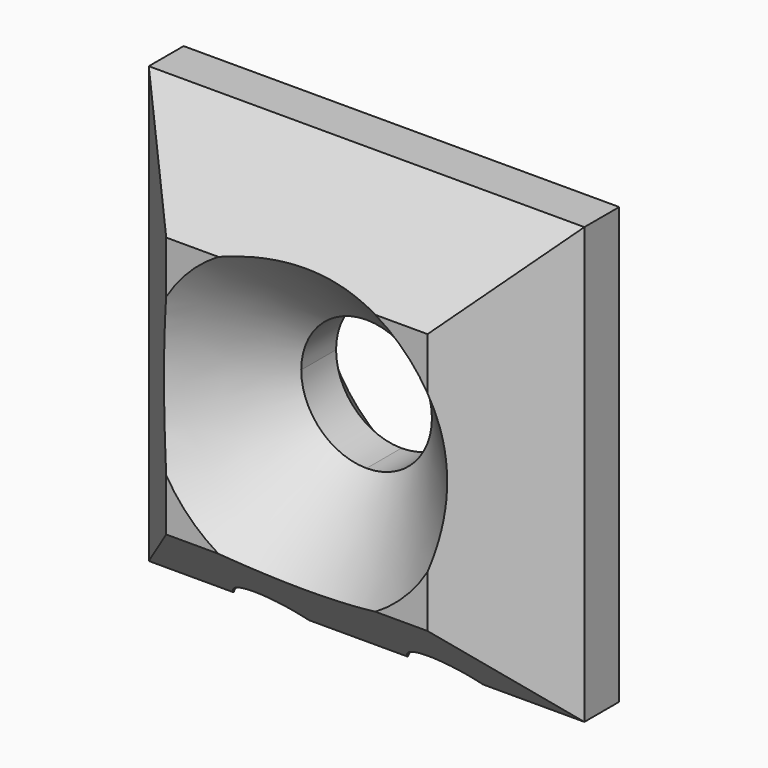
from build123d import *

# Parameters (mm, degrees)
F1_DEPTH    = 12.7
F2_R        = 2.54
F3_DEPTH    = 2.54
F4_T1_DEPTH = 51.5282991577
F4_T3_DEPTH = 51.5282991577


# Not quite as in the source:
# - a fillet or chamfer that OpenCascade refuses, or shapes differently, is made with other operations: its cross-section is extruded or revolved along the edge and cut away or added


with BuildPart() as f1:
    # F0 (on Front) → F1 (new body)
    with BuildSketch(Plane.XZ):
        with BuildLine():
            Line((0, 25.4), (0, 12.7))
            Line((0, 12.7), (8.89, 12.7))
            ThreePointArc((8.89, 12.7), (10.0059231637, 15.3940768363), (12.7, 16.51))
            Line((12.7, 16.51), (12.7, 25.4))
            Line((12.7, 25.4), (0, 25.4))
        make_face()
        with BuildLine():
            Line((16.51, 12.7), (25.4, 12.7))
            Line((25.4, 12.7), (25.4, 25.4))
            Line((25.4, 25.4), (12.7, 25.4))
            Line((12.7, 25.4), (12.7, 16.51))
            ThreePointArc((12.7, 16.51), (15.3940768363, 15.3940768363), (16.51, 12.7))
        make_face()
        with BuildLine():
            Line((12.7, 8.89), (12.7, 0))
            Line((12.7, 0), (25.4, 0))
            Line((25.4, 0), (25.4, 12.7))
            Line((25.4, 12.7), (16.51, 12.7))
            ThreePointArc((16.51, 12.7), (15.3940768363, 10.0059231637), (12.7, 8.89))
        make_face()
        with BuildLine():
            Line((0, 12.7), (0, 0))
            Line((0, 0), (12.7, 0))
            Line((12.7, 0), (12.7, 8.89))
            ThreePointArc((12.7, 8.89), (10.0059231637, 10.0059231637), (8.89, 12.7))
            Line((8.89, 12.7), (0, 12.7))
        make_face()
    extrude(amount=F1_DEPTH)

    # F2 (on Top) → F3 (cut)
    with BuildSketch(Plane.XY):
        with Locations((7.1409146445, -6.35)):
            Circle(F2_R)
        with Locations((17.3009146445, -6.35)):
            Circle(F2_R)
    extrude(amount=F3_DEPTH, mode=Mode.SUBTRACT)

    # F4: chamfer of 5.08 on 10 edges, made by hand

    # F4_s2 → F4_t1 (cut)
    with BuildSketch(Plane.XY.offset(-13.0641495789)):
        Polygon((0, -7.62), (5.08, -12.7), (0, -12.7), align=None)
        Polygon((20.32, -12.7), (25.4, -7.62), (25.4, -12.7), align=None)
        Polygon((0, -5.08), (5.08, 0), (0, 0), align=None)
        Polygon((20.32, 0), (25.4, -5.08), (25.4, 0), align=None)
    extrude(amount=F4_T1_DEPTH, mode=Mode.SUBTRACT)

    # F4_s4 → F4_t3 (cut)
    with BuildSketch(Plane.YZ.offset(-13.0641495789)):
        Polygon((-7.62, 0), (-12.7, 5.08), (-12.7, 0), align=None)
        Polygon((-7.62, 25.4), (-12.7, 20.32), (-12.7, 25.4), align=None)
        Polygon((-5.08, 0), (0, 5.08), (0, 0), align=None)
        Polygon((-5.08, 25.4), (0, 20.32), (0, 25.4), align=None)
    extrude(amount=F4_T3_DEPTH, mode=Mode.SUBTRACT)

    # F4_s5 → F4_t6 (revolve, cut)
    with BuildSketch(Plane.YZ.offset(12.7)):
        Polygon((-12.7, 3.81), (-7.62, 8.89), (-12.7, 8.89), align=None)
    revolve(axis=Axis((12.7, -12.7, 12.7), (0, 1, 0)), mode=Mode.SUBTRACT)

    # F4_s7 → F4_t8 (revolve, cut)
    with BuildSketch(Plane.YZ.offset(12.7)):
        Polygon((0, 3.81), (-5.08, 8.89), (0, 8.89), align=None)
    revolve(axis=Axis((12.7, 0, 12.7), (0, 1, 0)), mode=Mode.SUBTRACT)


solid = f1.part
